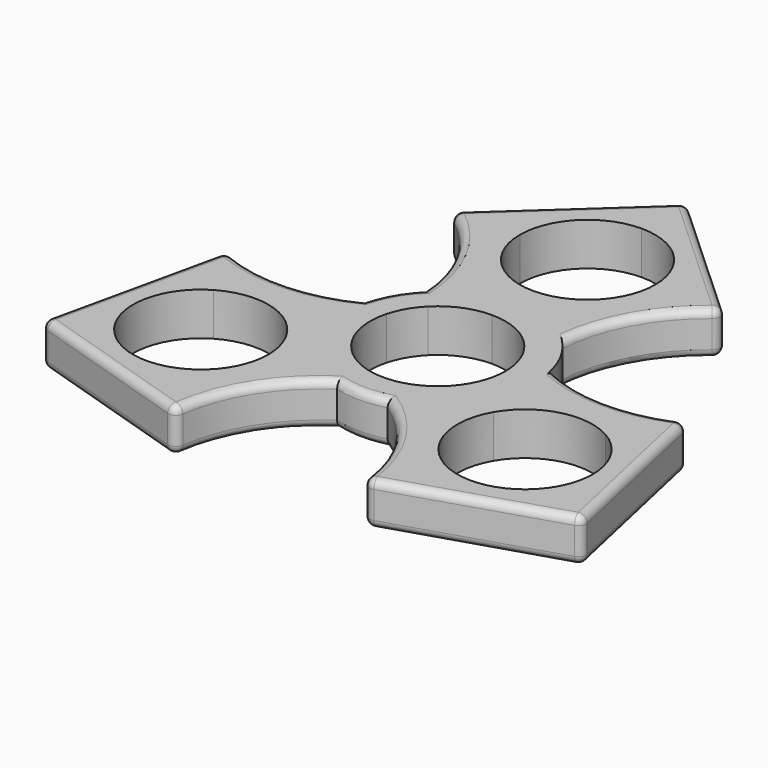
from build123d import *

# Parameters (mm, degrees)
F1_DEPTH      = 6.985
F2_R          = 1.27
F3_T3_DEPTH   = 27.3566440137
F3_T6_ANGLE   = 55.4439181523
F3_S7_R       = 15.875
F3_T8_DEPTH   = 16
F3_T11_DEPTH  = 27.3566440137
F3_T14_DEPTH  = 27.3566440137
F3_T17_ANGLE  = 55.4439181523
F3_S18_R      = 15.875
F3_T19_DEPTH  = 16
F3_T22_ANGLE  = 52.919334491
F3_S23_R      = 25.4
F3_T24_DEPTH  = 10
F3_S25_R      = 25.4
F3_T26_DEPTH  = 10
F3_T29_ANGLE  = 55.4439181523
F3_S30_R      = 15.875
F3_T31_DEPTH  = 15
F3_T34_DEPTH  = 27.3566440137
F3_T37_ANGLE  = 55.4439181523
F3_S38_R      = 15.875
F3_T39_DEPTH  = 16
F3_T42_ANGLE  = 55.4439181523
F3_S43_R      = 15.875
F3_T44_DEPTH  = 15
F3_T47_DEPTH  = 27.3566440137
F3_T50_DEPTH  = 27.3566440137
F3_T53_ANGLE  = 55.4439181523
F3_S54_R      = 15.875
F3_T55_DEPTH  = 16
F3_T58_ANGLE  = 52.919334491
F3_S59_R      = 25.4
F3_T60_DEPTH  = 9
F3_S61_R      = 25.4
F3_T62_DEPTH  = 9
F3_T65_DEPTH  = 27.3566440137
F3_T68_DEPTH  = 27.3566440137
F3_T71_ANGLE  = 55.4439181523
F3_S72_R      = 15.875
F3_T73_DEPTH  = 16
F3_T76_ANGLE  = 52.919334491
F3_S77_R      = 25.4
F3_T78_DEPTH  = 10
F3_S79_R      = 25.4
F3_T80_DEPTH  = 10
F3_T83_ANGLE  = 55.4439181523
F3_S84_R      = 15.875
F3_T85_DEPTH  = 15
F3_T88_DEPTH  = 27.3566440137
F3_T91_DEPTH  = 27.3566440137
F3_T94_ANGLE  = 55.4439181523
F3_S95_R      = 15.875
F3_T96_DEPTH  = 16
F3_T99_ANGLE  = 52.919334491
F3_S100_R     = 25.4
F3_T101_DEPTH = 10
F3_S102_R     = 25.4
F3_T103_DEPTH = 10
F3_T106_ANGLE = 55.4439181523
F3_S107_R     = 15.875
F3_T108_DEPTH = 15
F3_T111_DEPTH = 27.3566440137
F3_T114_DEPTH = 27.3566440137
F3_T117_ANGLE = 55.4439181523
F3_S118_R     = 15.875
F3_T119_DEPTH = 16
F3_T122_ANGLE = 52.919334491
F3_S123_R     = 25.4
F3_T124_DEPTH = 9
F3_S125_R     = 25.4
F3_T126_DEPTH = 9
F3_T129_ANGLE = 55.4439181523
F3_S130_R     = 15.875
F3_T131_DEPTH = 16
F3_T134_ANGLE = 99.5162059051
F3_T137_ANGLE = 99.5162059051
F3_T140_ANGLE = 85.0357607308
F3_T143_ANGLE = 99.5162059051
F3_T146_ANGLE = 99.5162059051
F3_T149_ANGLE = 85.0357607308
F3_T152_ANGLE = 99.5162059051
F3_T155_ANGLE = 99.5162059051
F3_T158_ANGLE = 85.0357607308
F3_T161_ANGLE = 99.5162059051
F3_T164_ANGLE = 85.0357607308
F3_T167_ANGLE = 99.5162059051
F3_T170_ANGLE = 99.5162059051
F3_T173_ANGLE = 85.0357607308
F3_T176_ANGLE = 99.5162059051
F3_T179_ANGLE = 99.5162059051
F3_T182_ANGLE = 85.0357607308
F3_T185_ANGLE = 99.5162059051
F3_T189_ANGLE = 52.919334491
F3_S190_R     = 25.4
F3_T191_DEPTH = 9
F3_T194_ANGLE = 55.4439181523
F3_S195_R     = 15.875
F3_T196_DEPTH = 16
F3_T201_ANGLE = 52.919334491
F3_S202_R     = 25.4
F3_T203_DEPTH = 10
F3_T206_ANGLE = 55.4439181523
F3_S207_R     = 15.875
F3_T208_DEPTH = 16
F3_T213_ANGLE = 55.4439181523
F3_S214_R     = 15.875
F3_T215_DEPTH = 15
F3_T218_ANGLE = 52.919334491
F3_S219_R     = 25.4
F3_T220_DEPTH = 10
F3_T225_ANGLE = 55.4439181523
F3_S226_R     = 15.875
F3_T227_DEPTH = 16
F3_T230_ANGLE = 52.919334491
F3_S231_R     = 25.4
F3_T232_DEPTH = 9
F3_T237_ANGLE = 52.919334491
F3_S238_R     = 25.4
F3_T239_DEPTH = 10
F3_T242_ANGLE = 55.4439181523
F3_S243_R     = 15.875
F3_T244_DEPTH = 16
F3_T249_ANGLE = 55.4439181523
F3_S250_R     = 15.875
F3_T251_DEPTH = 15
F3_T254_ANGLE = 52.919334491
F3_S255_R     = 25.4
F3_T256_DEPTH = 10
F3_T261_ANGLE = 52.919334491
F3_S262_R     = 25.4
F3_T263_DEPTH = 10
F3_T266_ANGLE = 55.4439181523
F3_S267_R     = 15.875
F3_T268_DEPTH = 16
F3_T273_ANGLE = 55.4439181523
F3_S274_R     = 15.875
F3_T275_DEPTH = 15
F3_T278_ANGLE = 52.919334491
F3_S279_R     = 25.4
F3_T280_DEPTH = 10
F3_T285_ANGLE = 55.4439181523
F3_S286_R     = 15.875
F3_T287_DEPTH = 16
F3_T290_ANGLE = 52.919334491
F3_S291_R     = 25.4
F3_T292_DEPTH = 9
F3_T297_ANGLE = 52.919334491
F3_S298_R     = 25.4
F3_T299_DEPTH = 9
F3_T302_ANGLE = 55.4439181523
F3_S303_R     = 15.875
F3_T304_DEPTH = 16


# Not quite as in the source:
# - a fillet or chamfer that OpenCascade refuses, or shapes differently, is made with other operations: its cross-section is extruded or revolved along the edge and cut away or added


with BuildPart() as f1:
    # F0 (on Top) → F1 (new body)
    with BuildSketch(Plane.XY):
        with BuildLine():
            ThreePointArc((10.6357126807, 2.8498306237), (10.9167002241, 1.4372108499), (11.0109, 0))
            ThreePointArc((11.0109, 0), (10.6357126807, -2.8498306237), (9.5357191185, -5.50545))
            Line((9.5357191185, -5.50545), (13.7481532851, -7.9375))
            ThreePointArc((13.7481532851, -7.9375), (15.3340724923, -4.108752341), (15.875, 0))
            ThreePointArc((15.875, 0), (15.7391871743, 2.0721033015), (15.3340724923, 4.108752341))
            Line((15.3340724923, 4.108752341), (10.6357126807, 2.8498306237))
        make_face()
        with BuildLine():
            ThreePointArc((7.785882057, 7.785882057), (9.5357191185, 5.50545), (10.6357126807, 2.8498306237))
            Line((10.6357126807, 2.8498306237), (15.3340724923, 4.108752341))
            ThreePointArc((15.3340724923, 4.108752341), (13.7481532851, 7.9375), (11.2253201513, 11.2253201513))
            Line((11.2253201513, 11.2253201513), (7.785882057, 7.785882057))
        make_face()
        with BuildLine():
            Line((13.7481532851, -7.9375), (9.5357191185, -5.50545))
            ThreePointArc((9.5357191185, -5.50545), (6.7030112187, -8.7355342946), (2.8498306237, -10.6357126807))
            Line((2.8498306237, -10.6357126807), (4.108752341, -15.3340724923))
            ThreePointArc((4.108752341, -15.3340724923), (9.6640876855, -12.5944842771), (13.7481532851, -7.9375))
        make_face()
        with BuildLine():
            ThreePointArc((0, 11.0109), (4.2136890054, 10.1727451445), (7.785882057, 7.785882057))
            Line((7.785882057, 7.785882057), (11.2253201513, 11.2253201513))
            ThreePointArc((11.2253201513, 11.2253201513), (6.0750994888, 14.6665875786), (0, 15.875))
            Line((0, 15.875), (0, 11.0109))
        make_face()
        with BuildLine():
            ThreePointArc((37.4772043073, 3.952421986), (26.387705649, 1.4905349479), (15.3340724923, 4.108752341))
            ThreePointArc((15.3340724923, 4.108752341), (15.7391871743, 2.0721033015), (15.875, 0))
            ThreePointArc((15.875, 0), (15.3340724923, -4.108752341), (13.7481532851, -7.9375))
            Line((13.7481532851, -7.9375), (16.8607351888, -9.73455))
            ThreePointArc((16.8607351888, -9.73455), (23.5466236836, -4.6042873193), (31.9019043073, -5.7042808815))
            Line((31.9019043073, -5.7042808815), (37.4772043073, 3.952421986))
        make_face()
        with BuildLine():
            Line((4.108752341, -15.3340724923), (2.8498306237, -10.6357126807))
            ThreePointArc((2.8498306237, -10.6357126807), (0, -11.0109), (-2.8498306237, -10.6357126807))
            Line((-2.8498306237, -10.6357126807), (-4.108752341, -15.3340724923))
            ThreePointArc((-4.108752341, -15.3340724923), (0, -15.875), (4.108752341, -15.3340724923))
        make_face()
        with BuildLine():
            Line((16.8607351888, -9.73455), (13.7481532851, -7.9375))
            ThreePointArc((13.7481532851, -7.9375), (9.6640876855, -12.5944842771), (4.108752341, -15.3340724923))
            ThreePointArc((4.108752341, -15.3340724923), (11.9030116944, -23.5976909136), (15.3157043073, -34.432421986))
            Line((15.3157043073, -34.432421986), (20.8910043073, -24.7757191185))
            ThreePointArc((20.8910043073, -24.7757191185), (15.7607416267, -18.0898306237), (16.8607351888, -9.73455))
        make_face()
        with BuildLine():
            ThreePointArc((-7.785882057, 7.785882057), (-4.2136890054, 10.1727451445), (0, 11.0109))
            Line((0, 11.0109), (0, 15.875))
            ThreePointArc((0, 15.875), (-6.0750994888, 14.6665875786), (-11.2253201513, 11.2253201513))
            Line((-11.2253201513, 11.2253201513), (-7.785882057, 7.785882057))
        make_face()
        with BuildLine():
            ThreePointArc((0, 15.875), (6.0750994888, 14.6665875786), (11.2253201513, 11.2253201513))
            ThreePointArc((11.2253201513, 11.2253201513), (14.4846939546, 22.1071559657), (22.1615, 30.48))
            Line((22.1615, 30.48), (11.0109, 30.48))
            ThreePointArc((11.0109, 30.48), (7.785882057, 22.694117943), (0, 19.4691))
            Line((0, 19.4691), (0, 15.875))
        make_face()
        with BuildLine():
            Line((-13.7481532851, -7.9375), (-9.5357191185, -5.50545))
            ThreePointArc((-9.5357191185, -5.50545), (-10.9167002241, -1.4372108499), (-10.6357126807, 2.8498306237))
            Line((-10.6357126807, 2.8498306237), (-15.3340724923, 4.108752341))
            ThreePointArc((-15.3340724923, 4.108752341), (-15.7391871743, -2.0721033015), (-13.7481532851, -7.9375))
        make_face()
        with BuildLine():
            ThreePointArc((-2.8498306237, -10.6357126807), (-6.7030112187, -8.7355342946), (-9.5357191185, -5.50545))
            Line((-9.5357191185, -5.50545), (-13.7481532851, -7.9375))
            ThreePointArc((-13.7481532851, -7.9375), (-9.6640876855, -12.5944842771), (-4.108752341, -15.3340724923))
            Line((-4.108752341, -15.3340724923), (-2.8498306237, -10.6357126807))
        make_face()
        with BuildLine():
            ThreePointArc((-10.6357126807, 2.8498306237), (-9.5357191185, 5.50545), (-7.785882057, 7.785882057))
            Line((-7.785882057, 7.785882057), (-11.2253201513, 11.2253201513))
            ThreePointArc((-11.2253201513, 11.2253201513), (-13.7481532851, 7.9375), (-15.3340724923, 4.108752341))
            Line((-15.3340724923, 4.108752341), (-10.6357126807, 2.8498306237))
        make_face()
        with BuildLine():
            Line((43.9940905122, -25.4), (37.4772043073, 3.952421986))
            Line((37.4772043073, 3.952421986), (31.9019043073, -5.7042808815))
            ThreePointArc((31.9019043073, -5.7042808815), (35.9321734259, -9.73455), (37.4073543073, -15.24))
            ThreePointArc((37.4073543073, -15.24), (37.032166988, -18.0898306237), (35.9321734259, -20.74545))
            Line((35.9321734259, -20.74545), (43.9940905122, -25.4))
        make_face()
        with BuildLine():
            ThreePointArc((-11.2253201513, 11.2253201513), (-6.0750994888, 14.6665875786), (0, 15.875))
            Line((0, 15.875), (0, 19.4691))
            ThreePointArc((0, 19.4691), (-7.785882057, 22.694117943), (-11.0109, 30.48))
            Line((-11.0109, 30.48), (-22.1615, 30.48))
            ThreePointArc((-22.1615, 30.48), (-14.4846939546, 22.1071559657), (-11.2253201513, 11.2253201513))
        make_face()
        with BuildLine():
            Line((11.0109, 30.48), (22.1615, 30.48))
            Line((22.1615, 30.48), (0, 50.8))
            Line((0, 50.8), (0, 41.4909))
            ThreePointArc((0, 41.4909), (7.785882057, 38.265882057), (11.0109, 30.48))
        make_face()
        with BuildLine():
            ThreePointArc((-4.108752341, -15.3340724923), (-9.6640876855, -12.5944842771), (-13.7481532851, -7.9375))
            Line((-13.7481532851, -7.9375), (-16.8607351888, -9.73455))
            ThreePointArc((-16.8607351888, -9.73455), (-15.7607416267, -12.3901693763), (-15.3855543073, -15.24))
            ThreePointArc((-15.3855543073, -15.24), (-16.8607351888, -20.74545), (-20.8910043073, -24.7757191185))
            Line((-20.8910043073, -24.7757191185), (-15.3157043073, -34.432421986))
            ThreePointArc((-15.3157043073, -34.432421986), (-11.9030116944, -23.5976909136), (-4.108752341, -15.3340724923))
        make_face()
        with BuildLine():
            Line((-16.8607351888, -9.73455), (-13.7481532851, -7.9375))
            ThreePointArc((-13.7481532851, -7.9375), (-15.7391871743, -2.0721033015), (-15.3340724923, 4.108752341))
            ThreePointArc((-15.3340724923, 4.108752341), (-26.387705649, 1.4905349479), (-37.4772043073, 3.952421986))
            Line((-37.4772043073, 3.952421986), (-31.9019043073, -5.7042808815))
            ThreePointArc((-31.9019043073, -5.7042808815), (-23.5466236836, -4.6042873193), (-16.8607351888, -9.73455))
        make_face()
        with BuildLine():
            Line((15.3157043073, -34.432421986), (43.9940905122, -25.4))
            Line((43.9940905122, -25.4), (35.9321734259, -20.74545))
            ThreePointArc((35.9321734259, -20.74545), (29.2462849311, -25.8757126807), (20.8910043073, -24.7757191185))
            Line((20.8910043073, -24.7757191185), (15.3157043073, -34.432421986))
        make_face()
        with BuildLine():
            Line((0, 41.4909), (0, 50.8))
            Line((0, 50.8), (-22.1615, 30.48))
            Line((-22.1615, 30.48), (-11.0109, 30.48))
            ThreePointArc((-11.0109, 30.48), (-7.785882057, 38.265882057), (0, 41.4909))
        make_face()
        with BuildLine():
            Line((-31.9019043073, -5.7042808815), (-37.4772043073, 3.952421986))
            Line((-37.4772043073, 3.952421986), (-43.9940905122, -25.4))
            Line((-43.9940905122, -25.4), (-35.9321734259, -20.74545))
            ThreePointArc((-35.9321734259, -20.74545), (-37.032166988, -12.3901693763), (-31.9019043073, -5.7042808815))
        make_face()
        with BuildLine():
            Line((-43.9940905122, -25.4), (-15.3157043073, -34.432421986))
            Line((-15.3157043073, -34.432421986), (-20.8910043073, -24.7757191185))
            ThreePointArc((-20.8910043073, -24.7757191185), (-29.2462849311, -25.8757126807), (-35.9321734259, -20.74545))
            Line((-35.9321734259, -20.74545), (-43.9940905122, -25.4))
        make_face()
    extrude(amount=F1_DEPTH)

    # F2
    f2_edges = [f1.edges().sort_by_distance(p)[0] for p in [
        (22.1615, 30.48, 3.4925),
        (0, 50.8, 3.4925),
        (-22.1615, 30.48, 3.4925),
        (37.477204, 3.952422, 3.4925),
        (43.994091, -25.4, 3.4925),
        (15.315704, -34.432422, 3.4925),
        (-15.315704, -34.432422, 3.4925),
        (-43.994091, -25.4, 3.4925),
        (-37.477204, 3.952422, 3.4925),
    ]]
    fillet(f2_edges, radius=F2_R)

    # F3: fillet of radius 1.27 on 29 edges, made by hand


with BuildPart() as f3_tool1:
    # F3_s2 → F3_t3 (new body)
    with BuildSketch(Plane(origin=(24.4464303747, 22.4150651, 0), x_dir=(0, 0, 1), z_dir=(-0.7370664686, -0.6758202578, 0))):
        with BuildLine():
            ThreePointArc((6.985, 36.1729766066), (6.6130256121, 37.0710022187), (5.715, 37.4429766066))
            Line((5.715, 37.4429766066), (6.985, 37.4429766066))
            Line((6.985, 37.4429766066), (6.985, 36.1729766066))
        make_face()
    extrude(amount=F3_T3_DEPTH)


with BuildPart() as f3_tool4:
    # F3_s5 → F3_t6 (revolve)
    with BuildSketch(Plane(origin=(-4.8108803435, -34.3795852428, 0), x_dir=(0, 0, 1), z_dir=(-0.1385839484, -0.99035069, 0))):
        with BuildLine():
            ThreePointArc((6.985, 11.7109494398), (6.6130256121, 10.8129238277), (5.715, 10.4409494398))
            Line((5.715, 10.4409494398), (6.985, 10.4409494398))
            Line((6.985, 10.4409494398), (6.985, 11.7109494398))
        make_face()
    revolve(axis=Axis((10.003825701, -36.452669534, 6.985), (0, 0, -1)), revolution_arc=F3_T6_ANGLE)

    # F3_s7 → F3_t8 (cut, symmetric)
    with BuildSketch(Plane.XY.offset(6.3)):
        Circle(F3_S7_R)
    extrude(amount=F3_T8_DEPTH, both=True, mode=Mode.SUBTRACT)


with BuildPart() as f3_tool9:
    # F3_s10 → F3_t11 (new body)
    with BuildSketch(Plane(origin=(-31.6352309914, 9.9636971863, 0), x_dir=(0, 0, 1), z_dir=(0.9538107459, -0.3004081572, 0))):
        with BuildLine():
            ThreePointArc((6.985, 36.1729766066), (6.6130256121, 37.0710022187), (5.715, 37.4429766066))
            Line((5.715, 37.4429766066), (6.985, 37.4429766066))
            Line((6.985, 37.4429766066), (6.985, 36.1729766066))
        make_face()
    extrude(amount=F3_T11_DEPTH)


with BuildPart() as f3_tool12:
    # F3_s13 → F3_t14 (new body)
    with BuildSketch(Plane(origin=(-1.2594045804, -5.672429061, 0), x_dir=(0, 0, 1), z_dir=(-0.2167442773, -0.976228415, 0))):
        with BuildLine():
            ThreePointArc((6.985, 36.1729766066), (6.6130256121, 37.0710022187), (5.715, 37.4429766066))
            Line((5.715, 37.4429766066), (6.985, 37.4429766066))
            Line((6.985, 37.4429766066), (6.985, 36.1729766066))
        make_face()
    extrude(amount=F3_T14_DEPTH)


with BuildPart() as f3_tool15:
    # F3_s16 → F3_t17 (revolve)
    with BuildSketch(Plane(origin=(-6.1527076501, -4.0584782097, 0), x_dir=(0, 0, 1), z_dir=(0.8347533892, 0.5506239908, 0))):
        with BuildLine():
            ThreePointArc((6.985, -10.4048781253), (6.6130256121, -11.3029037374), (5.715, -11.6748781253))
            Line((5.715, -11.6748781253), (6.985, -11.6748781253))
            Line((6.985, -11.6748781253), (6.985, -10.4048781253))
        make_face()
    revolve(axis=Axis((-26.5670250017, 26.8899019591, 6.985), (0, 0, -1)), revolution_arc=F3_T17_ANGLE)

    # F3_s18 → F3_t19 (cut, symmetric)
    with BuildSketch(Plane.XY.offset(6.3)):
        Circle(F3_S18_R)
    extrude(amount=F3_T19_DEPTH, both=True, mode=Mode.SUBTRACT)


with BuildPart() as f3_tool20:
    # F3_s21 → F3_t22 (revolve)
    with BuildSketch(Plane(origin=(0, 0, 0), x_dir=(0, 0, 1), z_dir=(0.8334970853, 0.5525238536, 0))):
        with BuildLine():
            ThreePointArc((6.985, -14.605), (6.6130256121, -15.5030256121), (5.715, -15.875))
            Line((5.715, -15.875), (6.985, -15.875))
            Line((6.985, -15.875), (6.985, -14.605))
        make_face()
    revolve(axis=Axis((0, 0, 6.985), (0, 0, 1)), revolution_arc=F3_T22_ANGLE)

    # F3_s23 → F3_t24 (intersect, symmetric)
    with BuildSketch(Plane.XY.offset(5.9)):
        with Locations((-36.5708507027, 9.5627675749)):
            Circle(F3_S23_R)
    extrude(amount=F3_T24_DEPTH, both=True, mode=Mode.INTERSECT)

    # F3_s25 → F3_t26 (intersect, symmetric)
    with BuildSketch(Plane.XY.offset(5.9)):
        with Locations((-26.5670250017, 26.8899019591)):
            Circle(F3_S25_R)
    extrude(amount=F3_T26_DEPTH, both=True, mode=Mode.INTERSECT)


with BuildPart() as f3_tool27:
    # F3_s28 → F3_t29 (revolve)
    with BuildSketch(Plane(origin=(-27.3681540201, 21.3561372134, 0), x_dir=(0, 0, 1), z_dir=(-0.788376882, 0.6151925649, 0))):
        with BuildLine():
            ThreePointArc((6.985, 11.7109494398), (6.6130256121, 10.8129238277), (5.715, 10.4409494398))
            Line((5.715, 10.4409494398), (6.985, 10.4409494398))
            Line((6.985, 10.4409494398), (6.985, 11.7109494398))
        make_face()
    revolve(axis=Axis((-36.5708507027, 9.5627675749, 6.985), (0, 0, -1)), revolution_arc=F3_T29_ANGLE)

    # F3_s30 → F3_t31 (cut, symmetric)
    with BuildSketch(Plane.XY.offset(5.9)):
        Circle(F3_S30_R)
    extrude(amount=F3_T31_DEPTH, both=True, mode=Mode.SUBTRACT)


with BuildPart() as f3_tool32:
    # F3_s33 → F3_t34 (new body)
    with BuildSketch(Plane(origin=(-4.2827653778, 3.9268908908, 0), x_dir=(0, 0, 1), z_dir=(-0.7370664686, 0.6758202578, 0))):
        with BuildLine():
            ThreePointArc((6.985, 36.1729766066), (6.6130256121, 37.0710022187), (5.715, 37.4429766066))
            Line((5.715, 37.4429766066), (6.985, 37.4429766066))
            Line((6.985, 37.4429766066), (6.985, 36.1729766066))
        make_face()
    extrude(amount=F3_T34_DEPTH)


with BuildPart() as f3_tool35:
    # F3_s36 → F3_t37 (revolve)
    with BuildSketch(Plane(origin=(-0.4383914053, 7.3576402319, 0), x_dir=(0, 0, 1), z_dir=(0.0594776694, -0.9982296363, 0))):
        with BuildLine():
            ThreePointArc((6.985, -10.4048781253), (6.6130256121, -11.3029037374), (5.715, -11.6748781253))
            Line((5.715, -11.6748781253), (6.985, -11.6748781253))
            Line((6.985, -11.6748781253), (6.985, -10.4048781253))
        make_face()
    revolve(axis=Axis((36.5708507027, 9.5627675749, 6.985), (0, 0, -1)), revolution_arc=F3_T37_ANGLE)

    # F3_s38 → F3_t39 (cut, symmetric)
    with BuildSketch(Plane.XY.offset(6.3)):
        Circle(F3_S38_R)
    extrude(amount=F3_T39_DEPTH, both=True, mode=Mode.SUBTRACT)


with BuildPart() as f3_tool40:
    # F3_s41 → F3_t42 (revolve)
    with BuildSketch(Plane(origin=(32.1790343636, 13.0234480294, 0), x_dir=(0, 0, 1), z_dir=(0.9269608304, 0.3751581251, 0))):
        with BuildLine():
            ThreePointArc((5.715, 10.4409494398), (6.6130256121, 10.8129238277), (6.985, 11.7109494398))
            Line((6.985, 11.7109494398), (6.985, 10.4409494398))
            Line((6.985, 10.4409494398), (5.715, 10.4409494398))
        make_face()
    revolve(axis=Axis((26.5670250017, 26.8899019591, 6.985), (0, 0, -1)), revolution_arc=F3_T42_ANGLE)

    # F3_s43 → F3_t44 (cut, symmetric)
    with BuildSketch(Plane.XY.offset(5.9)):
        Circle(F3_S43_R)
    extrude(amount=F3_T44_DEPTH, both=True, mode=Mode.SUBTRACT)


with BuildPart() as f3_tool45:
    # F3_s46 → F3_t47 (new body)
    with BuildSketch(Plane(origin=(7.1888006167, -32.3787622863, 0), x_dir=(0, 0, 1), z_dir=(-0.2167442773, 0.976228415, 0))):
        with BuildLine():
            ThreePointArc((6.985, 36.1729766066), (6.6130256121, 37.0710022187), (5.715, 37.4429766066))
            Line((5.715, 37.4429766066), (6.985, 37.4429766066))
            Line((6.985, 37.4429766066), (6.985, 36.1729766066))
        make_face()
    extrude(amount=F3_T47_DEPTH)


with BuildPart() as f3_tool48:
    # F3_s49 → F3_t50 (new body)
    with BuildSketch(Plane(origin=(5.5421699582, 1.7455381702, 0), x_dir=(0, 0, 1), z_dir=(0.9538107459, 0.3004081572, 0))):
        with BuildLine():
            ThreePointArc((6.985, 36.1729766066), (6.6130256121, 37.0710022187), (5.715, 37.4429766066))
            Line((5.715, 37.4429766066), (6.985, 37.4429766066))
            Line((6.985, 37.4429766066), (6.985, 36.1729766066))
        make_face()
    extrude(amount=F3_T50_DEPTH)


with BuildPart() as f3_tool51:
    # F3_s52 → F3_t53 (revolve)
    with BuildSketch(Plane(origin=(6.5910990554, -3.2991620222, 0), x_dir=(0, 0, 1), z_dir=(-0.8942310586, 0.4476056455, 0))):
        with BuildLine():
            ThreePointArc((6.985, -10.4048781253), (6.6130256121, -11.3029037374), (5.715, -11.6748781253))
            Line((5.715, -11.6748781253), (6.985, -11.6748781253))
            Line((6.985, -11.6748781253), (6.985, -10.4048781253))
        make_face()
    revolve(axis=Axis((-10.003825701, -36.452669534, 6.985), (0, 0, -1)), revolution_arc=F3_T53_ANGLE)

    # F3_s54 → F3_t55 (cut, symmetric)
    with BuildSketch(Plane.XY.offset(5.9)):
        Circle(F3_S54_R)
    extrude(amount=F3_T55_DEPTH, both=True, mode=Mode.SUBTRACT)


with BuildPart() as f3_tool56:
    # F3_s57 → F3_t58 (revolve)
    with BuildSketch(Plane(origin=(0, 0, 0), x_dir=(0, 0, 1), z_dir=(-0.895248236, 0.4455677231, 0))):
        with BuildLine():
            ThreePointArc((6.985, -14.605), (6.6130256121, -15.5030256121), (5.715, -15.875))
            Line((5.715, -15.875), (6.985, -15.875))
            Line((6.985, -15.875), (6.985, -14.605))
        make_face()
    revolve(axis=Axis((0, 0, 6.985), (0, 0, 1)), revolution_arc=F3_T58_ANGLE)

    # F3_s59 → F3_t60 (intersect, symmetric)
    with BuildSketch(Plane.XY.offset(5.9)):
        with Locations((-10.003825701, -36.452669534)):
            Circle(F3_S59_R)
    extrude(amount=F3_T60_DEPTH, both=True, mode=Mode.INTERSECT)

    # F3_s61 → F3_t62 (intersect, symmetric)
    with BuildSketch(Plane.XY.offset(5.9)):
        with Locations((10.003825701, -36.452669534)):
            Circle(F3_S61_R)
    extrude(amount=F3_T62_DEPTH, both=True, mode=Mode.INTERSECT)


with BuildPart() as f3_tool63:
    # F3_s64 → F3_t65 (new body)
    with BuildSketch(Plane(origin=(-31.6352309914, 9.9636971863, 0), x_dir=(0, 0, 1), z_dir=(0.9538107459, -0.3004081572, 0))):
        with BuildLine():
            ThreePointArc((0, 36.1729766066), (0.3719743879, 37.0710022187), (1.27, 37.4429766066))
            Line((1.27, 37.4429766066), (0, 37.4429766066))
            Line((0, 37.4429766066), (0, 36.1729766066))
        make_face()
    extrude(amount=F3_T65_DEPTH)


with BuildPart() as f3_tool66:
    # F3_s67 → F3_t68 (new body)
    with BuildSketch(Plane(origin=(-1.2594045804, -5.672429061, 0), x_dir=(0, 0, 1), z_dir=(-0.2167442773, -0.976228415, 0))):
        with BuildLine():
            ThreePointArc((0, 36.1729766066), (0.3719743879, 37.0710022187), (1.27, 37.4429766066))
            Line((1.27, 37.4429766066), (0, 37.4429766066))
            Line((0, 37.4429766066), (0, 36.1729766066))
        make_face()
    extrude(amount=F3_T68_DEPTH)


with BuildPart() as f3_tool69:
    # F3_s70 → F3_t71 (revolve)
    with BuildSketch(Plane(origin=(-6.1527076501, -4.0584782097, 0), x_dir=(0, 0, 1), z_dir=(0.8347533892, 0.5506239908, 0))):
        with BuildLine():
            ThreePointArc((0, -10.4048781253), (0.3719743879, -11.3029037374), (1.27, -11.6748781253))
            Line((1.27, -11.6748781253), (0, -11.6748781253))
            Line((0, -11.6748781253), (0, -10.4048781253))
        make_face()
    revolve(axis=Axis((-26.5670250017, 26.8899019591, 0), (0, 0, -1)), revolution_arc=F3_T71_ANGLE)

    # F3_s72 → F3_t73 (cut, symmetric)
    with BuildSketch(Plane.XY.offset(0.6)):
        Circle(F3_S72_R)
    extrude(amount=F3_T73_DEPTH, both=True, mode=Mode.SUBTRACT)


with BuildPart() as f3_tool74:
    # F3_s75 → F3_t76 (revolve)
    with BuildSketch(Plane(origin=(0, 0, 0), x_dir=(0, 0, 1), z_dir=(0.8334970853, 0.5525238536, 0))):
        with BuildLine():
            ThreePointArc((0, -14.605), (0.3719743879, -15.5030256121), (1.27, -15.875))
            Line((1.27, -15.875), (0, -15.875))
            Line((0, -15.875), (0, -14.605))
        make_face()
    revolve(axis=Axis((0, 0, 0), (0, 0, 1)), revolution_arc=F3_T76_ANGLE)

    # F3_s77 → F3_t78 (intersect, symmetric)
    with BuildSketch(Plane.XY.offset(1.1)):
        with Locations((-36.5708507027, 9.5627675749)):
            Circle(F3_S77_R)
    extrude(amount=F3_T78_DEPTH, both=True, mode=Mode.INTERSECT)

    # F3_s79 → F3_t80 (intersect, symmetric)
    with BuildSketch(Plane.XY.offset(1.1)):
        with Locations((-26.5670250017, 26.8899019591)):
            Circle(F3_S79_R)
    extrude(amount=F3_T80_DEPTH, both=True, mode=Mode.INTERSECT)


with BuildPart() as f3_tool81:
    # F3_s82 → F3_t83 (revolve)
    with BuildSketch(Plane(origin=(-27.3681540201, 21.3561372134, 0), x_dir=(0, 0, 1), z_dir=(-0.788376882, 0.6151925649, 0))):
        with BuildLine():
            ThreePointArc((0, 11.7109494398), (0.3719743879, 10.8129238277), (1.27, 10.4409494398))
            Line((1.27, 10.4409494398), (0, 10.4409494398))
            Line((0, 10.4409494398), (0, 11.7109494398))
        make_face()
    revolve(axis=Axis((-36.5708507027, 9.5627675749, 0), (0, 0, -1)), revolution_arc=F3_T83_ANGLE)

    # F3_s84 → F3_t85 (cut, symmetric)
    with BuildSketch(Plane.XY.offset(1.1)):
        Circle(F3_S84_R)
    extrude(amount=F3_T85_DEPTH, both=True, mode=Mode.SUBTRACT)


with BuildPart() as f3_tool86:
    # F3_s87 → F3_t88 (new body)
    with BuildSketch(Plane(origin=(24.4464303747, 22.4150651, 0), x_dir=(0, 0, 1), z_dir=(-0.7370664686, -0.6758202578, 0))):
        with BuildLine():
            ThreePointArc((0, 36.1729766066), (0.3719743879, 37.0710022187), (1.27, 37.4429766066))
            Line((1.27, 37.4429766066), (0, 37.4429766066))
            Line((0, 37.4429766066), (0, 36.1729766066))
        make_face()
    extrude(amount=F3_T88_DEPTH)


with BuildPart() as f3_tool89:
    # F3_s90 → F3_t91 (new body)
    with BuildSketch(Plane(origin=(-4.2827653778, 3.9268908908, 0), x_dir=(0, 0, 1), z_dir=(-0.7370664686, 0.6758202578, 0))):
        with BuildLine():
            ThreePointArc((0, 36.1729766066), (0.3719743879, 37.0710022187), (1.27, 37.4429766066))
            Line((1.27, 37.4429766066), (0, 37.4429766066))
            Line((0, 37.4429766066), (0, 36.1729766066))
        make_face()
    extrude(amount=F3_T91_DEPTH)


with BuildPart() as f3_tool92:
    # F3_s93 → F3_t94 (revolve)
    with BuildSketch(Plane(origin=(-0.4383914053, 7.3576402319, 0), x_dir=(0, 0, 1), z_dir=(0.0594776694, -0.9982296363, 0))):
        with BuildLine():
            ThreePointArc((0, -10.4048781253), (0.3719743879, -11.3029037374), (1.27, -11.6748781253))
            Line((1.27, -11.6748781253), (0, -11.6748781253))
            Line((0, -11.6748781253), (0, -10.4048781253))
        make_face()
    revolve(axis=Axis((36.5708507027, 9.5627675749, 0), (0, 0, -1)), revolution_arc=F3_T94_ANGLE)

    # F3_s95 → F3_t96 (cut, symmetric)
    with BuildSketch(Plane.XY.offset(0.6)):
        Circle(F3_S95_R)
    extrude(amount=F3_T96_DEPTH, both=True, mode=Mode.SUBTRACT)


with BuildPart() as f3_tool97:
    # F3_s98 → F3_t99 (revolve)
    with BuildSketch(Plane(origin=(0, 0, 0), x_dir=(0, 0, 1), z_dir=(0.0617511507, -0.9980915767, 0))):
        with BuildLine():
            ThreePointArc((0, -14.605), (0.3719743879, -15.5030256121), (1.27, -15.875))
            Line((1.27, -15.875), (0, -15.875))
            Line((0, -15.875), (0, -14.605))
        make_face()
    revolve(axis=Axis((0, 0, 0), (0, 0, 1)), revolution_arc=F3_T99_ANGLE)

    # F3_s100 → F3_t101 (intersect, symmetric)
    with BuildSketch(Plane.XY.offset(1.1)):
        with Locations((26.5670250017, 26.8899019591)):
            Circle(F3_S100_R)
    extrude(amount=F3_T101_DEPTH, both=True, mode=Mode.INTERSECT)

    # F3_s102 → F3_t103 (intersect, symmetric)
    with BuildSketch(Plane.XY.offset(1.1)):
        with Locations((36.5708507027, 9.5627675749)):
            Circle(F3_S102_R)
    extrude(amount=F3_T103_DEPTH, both=True, mode=Mode.INTERSECT)


with BuildPart() as f3_tool104:
    # F3_s105 → F3_t106 (revolve)
    with BuildSketch(Plane(origin=(32.1790343636, 13.0234480294, 0), x_dir=(0, 0, 1), z_dir=(0.9269608304, 0.3751581251, 0))):
        with BuildLine():
            ThreePointArc((1.27, 10.4409494398), (0.3719743879, 10.8129238277), (0, 11.7109494398))
            Line((0, 11.7109494398), (0, 10.4409494398))
            Line((0, 10.4409494398), (1.27, 10.4409494398))
        make_face()
    revolve(axis=Axis((26.5670250017, 26.8899019591, 0), (0, 0, -1)), revolution_arc=F3_T106_ANGLE)

    # F3_s107 → F3_t108 (cut, symmetric)
    with BuildSketch(Plane.XY.offset(1.1)):
        Circle(F3_S107_R)
    extrude(amount=F3_T108_DEPTH, both=True, mode=Mode.SUBTRACT)


with BuildPart() as f3_tool109:
    # F3_s110 → F3_t111 (new body)
    with BuildSketch(Plane(origin=(7.1888006167, -32.3787622863, 0), x_dir=(0, 0, 1), z_dir=(-0.2167442773, 0.976228415, 0))):
        with BuildLine():
            ThreePointArc((0, 36.1729766066), (0.3719743879, 37.0710022187), (1.27, 37.4429766066))
            Line((1.27, 37.4429766066), (0, 37.4429766066))
            Line((0, 37.4429766066), (0, 36.1729766066))
        make_face()
    extrude(amount=F3_T111_DEPTH)


with BuildPart() as f3_tool112:
    # F3_s113 → F3_t114 (new body)
    with BuildSketch(Plane(origin=(5.5421699582, 1.7455381702, 0), x_dir=(0, 0, 1), z_dir=(0.9538107459, 0.3004081572, 0))):
        with BuildLine():
            ThreePointArc((0, 36.1729766066), (0.3719743879, 37.0710022187), (1.27, 37.4429766066))
            Line((1.27, 37.4429766066), (0, 37.4429766066))
            Line((0, 37.4429766066), (0, 36.1729766066))
        make_face()
    extrude(amount=F3_T114_DEPTH)


with BuildPart() as f3_tool115:
    # F3_s116 → F3_t117 (revolve)
    with BuildSketch(Plane(origin=(6.5910990554, -3.2991620222, 0), x_dir=(0, 0, 1), z_dir=(-0.8942310586, 0.4476056455, 0))):
        with BuildLine():
            ThreePointArc((0, -10.4048781253), (0.3719743879, -11.3029037374), (1.27, -11.6748781253))
            Line((1.27, -11.6748781253), (0, -11.6748781253))
            Line((0, -11.6748781253), (0, -10.4048781253))
        make_face()
    revolve(axis=Axis((-10.003825701, -36.452669534, 0), (0, 0, -1)), revolution_arc=F3_T117_ANGLE)

    # F3_s118 → F3_t119 (cut, symmetric)
    with BuildSketch(Plane.XY.offset(1.1)):
        Circle(F3_S118_R)
    extrude(amount=F3_T119_DEPTH, both=True, mode=Mode.SUBTRACT)


with BuildPart() as f3_tool120:
    # F3_s121 → F3_t122 (revolve)
    with BuildSketch(Plane(origin=(0, 0, 0), x_dir=(0, 0, 1), z_dir=(-0.895248236, 0.4455677231, 0))):
        with BuildLine():
            ThreePointArc((0, -14.605), (0.3719743879, -15.5030256121), (1.27, -15.875))
            Line((1.27, -15.875), (0, -15.875))
            Line((0, -15.875), (0, -14.605))
        make_face()
    revolve(axis=Axis((0, 0, 0), (0, 0, 1)), revolution_arc=F3_T122_ANGLE)

    # F3_s123 → F3_t124 (intersect, symmetric)
    with BuildSketch(Plane.XY.offset(1.1)):
        with Locations((-10.003825701, -36.452669534)):
            Circle(F3_S123_R)
    extrude(amount=F3_T124_DEPTH, both=True, mode=Mode.INTERSECT)

    # F3_s125 → F3_t126 (intersect, symmetric)
    with BuildSketch(Plane.XY.offset(1.1)):
        with Locations((10.003825701, -36.452669534)):
            Circle(F3_S125_R)
    extrude(amount=F3_T126_DEPTH, both=True, mode=Mode.INTERSECT)


with BuildPart() as f3_tool127:
    # F3_s128 → F3_t129 (revolve)
    with BuildSketch(Plane(origin=(-4.8108803435, -34.3795852428, 0), x_dir=(0, 0, 1), z_dir=(-0.1385839484, -0.99035069, 0))):
        with BuildLine():
            ThreePointArc((0, 11.7109494398), (0.3719743879, 10.8129238277), (1.27, 10.4409494398))
            Line((1.27, 10.4409494398), (0, 10.4409494398))
            Line((0, 10.4409494398), (0, 11.7109494398))
        make_face()
    revolve(axis=Axis((10.003825701, -36.452669534, 0), (0, 0, -1)), revolution_arc=F3_T129_ANGLE)

    # F3_s130 → F3_t131 (cut, symmetric)
    with BuildSketch(Plane.XY.offset(0.6)):
        Circle(F3_S130_R)
    extrude(amount=F3_T131_DEPTH, both=True, mode=Mode.SUBTRACT)


with BuildPart() as f3_tool132:
    # F3_s133 → F3_t134 (revolve)
    with BuildSketch(Plane(origin=(-5.5421699582, 1.7455381702, 0), x_dir=(0, 0, 1), z_dir=(-0.9538107459, 0.3004081572, 0))):
        with BuildLine():
            ThreePointArc((0, -36.1729766066), (0.3719743879, -37.0710022187), (1.27, -37.4429766066))
            Line((1.27, -37.4429766066), (0, -37.4429766066))
            Line((0, -37.4429766066), (0, -36.1729766066))
        make_face()
    revolve(axis=Axis((-16.4088272021, -32.7566356298, 0), (0, 0, 1)), revolution_arc=F3_T134_ANGLE)


with BuildPart() as f3_tool135:
    # F3_s136 → F3_t137 (revolve)
    with BuildSketch(Plane(origin=(4.8108803435, -34.3795852428, 0), x_dir=(0, 0, 1), z_dir=(-0.1385839484, 0.99035069, 0))):
        with BuildLine():
            ThreePointArc((0, 11.7109494398), (0.3719743879, 10.8129238277), (1.27, 10.4409494398))
            Line((1.27, 10.4409494398), (0, 10.4409494398))
            Line((0, 10.4409494398), (0, 11.7109494398))
        make_face()
    revolve(axis=Axis((16.4088272021, -32.7566356298, 0), (0, 0, 1)), revolution_arc=F3_T137_ANGLE)


with BuildPart() as f3_tool138:
    # F3_s139 → F3_t140 (revolve)
    with BuildSketch(Plane(origin=(31.6352309914, 9.9636971863, 0), x_dir=(0, 0, 1), z_dir=(-0.9538107459, -0.3004081572, 0))):
        with BuildLine():
            ThreePointArc((0, -36.1729766066), (0.3719743879, -37.0710022187), (1.27, -37.4429766066))
            Line((1.27, -37.4429766066), (0, -37.4429766066))
            Line((0, -37.4429766066), (0, -36.1729766066))
        make_face()
    revolve(axis=Axis((42.5018882352, -24.5384766137, 0), (0, 0, 1)), revolution_arc=F3_T140_ANGLE)


with BuildPart() as f3_tool141:
    # F3_s142 → F3_t143 (revolve)
    with BuildSketch(Plane(origin=(32.1790343636, 13.0234480294, 0), x_dir=(0, 0, 1), z_dir=(-0.9269608304, -0.3751581251, 0))):
        with BuildLine():
            ThreePointArc((0, -11.7109494398), (0.3719743879, -10.8129238277), (1.27, -10.4409494398))
            Line((1.27, -10.4409494398), (0, -10.4409494398))
            Line((0, -10.4409494398), (0, -11.7109494398))
        make_face()
    revolve(axis=Axis((36.5724921989, 2.1678566116, 0), (0, 0, -1)), revolution_arc=F3_T143_ANGLE)


with BuildPart() as f3_tool144:
    # F3_s145 → F3_t146 (revolve)
    with BuildSketch(Plane(origin=(27.3681540201, 21.3561372134, 0), x_dir=(0, 0, 1), z_dir=(-0.788376882, -0.6151925649, 0))):
        with BuildLine():
            ThreePointArc((0, 11.7109494398), (0.3719743879, 10.8129238277), (1.27, 10.4409494398))
            Line((1.27, 10.4409494398), (0, 10.4409494398))
            Line((0, 10.4409494398), (0, 11.7109494398))
        make_face()
    revolve(axis=Axis((20.1636649969, 30.5887790182, 0), (0, 0, 1)), revolution_arc=F3_T146_ANGLE)


with BuildPart() as f3_tool147:
    # F3_s148 → F3_t149 (revolve)
    with BuildSketch(Plane(origin=(-24.4464303747, 22.4150651, 0), x_dir=(0, 0, 1), z_dir=(0.7370664686, -0.6758202578, 0))):
        with BuildLine():
            ThreePointArc((0, -36.1729766066), (0.3719743879, -37.0710022187), (1.27, -37.4429766066))
            Line((1.27, -37.4429766066), (0, -37.4429766066))
            Line((0, -37.4429766066), (0, -36.1729766066))
        make_face()
    revolve(axis=Axis((0, 49.0769532274, 0), (0, 0, 1)), revolution_arc=F3_T149_ANGLE)


with BuildPart() as f3_tool150:
    # F3_s151 → F3_t152 (revolve)
    with BuildSketch(Plane(origin=(4.2827653778, 3.9268908908, 0), x_dir=(0, 0, 1), z_dir=(0.7370664686, 0.6758202578, 0))):
        with BuildLine():
            ThreePointArc((0, -36.1729766066), (0.3719743879, -37.0710022187), (1.27, -37.4429766066))
            Line((1.27, -37.4429766066), (0, -37.4429766066))
            Line((0, -37.4429766066), (0, -36.1729766066))
        make_face()
    revolve(axis=Axis((-20.1636649969, 30.5887790182, 0), (0, 0, 1)), revolution_arc=F3_T152_ANGLE)


with BuildPart() as f3_tool153:
    # F3_s154 → F3_t155 (revolve)
    with BuildSketch(Plane(origin=(-32.1790343636, 13.0234480294, 0), x_dir=(0, 0, 1), z_dir=(0.9269608304, -0.3751581251, 0))):
        with BuildLine():
            ThreePointArc((0, 11.7109494398), (0.3719743879, 10.8129238277), (1.27, 10.4409494398))
            Line((1.27, 10.4409494398), (0, 10.4409494398))
            Line((0, 10.4409494398), (0, 11.7109494398))
        make_face()
    revolve(axis=Axis((-36.5724921989, 2.1678566116, 0), (0, 0, 1)), revolution_arc=F3_T155_ANGLE)


with BuildPart() as f3_tool156:
    # F3_s157 → F3_t158 (revolve)
    with BuildSketch(Plane(origin=(-7.1888006167, -32.3787622863, 0), x_dir=(0, 0, 1), z_dir=(0.2167442773, 0.976228415, 0))):
        with BuildLine():
            ThreePointArc((0, -36.1729766066), (0.3719743879, -37.0710022187), (1.27, -37.4429766066))
            Line((1.27, -37.4429766066), (0, -37.4429766066))
            Line((0, -37.4429766066), (0, -36.1729766066))
        make_face()
    revolve(axis=Axis((-42.5018882352, -24.5384766137, 0), (0, 0, 1)), revolution_arc=F3_T158_ANGLE)


with BuildPart() as f3_tool159:
    # F3_s160 → F3_t161 (revolve)
    with BuildSketch(Plane(origin=(4.8108803435, -34.3795852428, 0), x_dir=(0, 0, 1), z_dir=(-0.1385839484, 0.99035069, 0))):
        with BuildLine():
            ThreePointArc((6.985, 11.7109494398), (6.6130256121, 10.8129238277), (5.715, 10.4409494398))
            Line((5.715, 10.4409494398), (6.985, 10.4409494398))
            Line((6.985, 10.4409494398), (6.985, 11.7109494398))
        make_face()
    revolve(axis=Axis((16.4088272021, -32.7566356298, 6.985), (0, 0, 1)), revolution_arc=F3_T161_ANGLE)


with BuildPart() as f3_tool162:
    # F3_s163 → F3_t164 (revolve)
    with BuildSketch(Plane(origin=(31.6352309914, 9.9636971863, 0), x_dir=(0, 0, 1), z_dir=(-0.9538107459, -0.3004081572, 0))):
        with BuildLine():
            ThreePointArc((6.985, -36.1729766066), (6.6130256121, -37.0710022187), (5.715, -37.4429766066))
            Line((5.715, -37.4429766066), (6.985, -37.4429766066))
            Line((6.985, -37.4429766066), (6.985, -36.1729766066))
        make_face()
    revolve(axis=Axis((42.5018882352, -24.5384766137, 6.985), (0, 0, 1)), revolution_arc=F3_T164_ANGLE)


with BuildPart() as f3_tool165:
    # F3_s166 → F3_t167 (revolve)
    with BuildSketch(Plane(origin=(32.1790343636, 13.0234480294, 0), x_dir=(0, 0, 1), z_dir=(-0.9269608304, -0.3751581251, 0))):
        with BuildLine():
            ThreePointArc((5.715, -10.4409494398), (6.6130256121, -10.8129238277), (6.985, -11.7109494398))
            Line((6.985, -11.7109494398), (6.985, -10.4409494398))
            Line((6.985, -10.4409494398), (5.715, -10.4409494398))
        make_face()
    revolve(axis=Axis((36.5724921989, 2.1678566116, 6.985), (0, 0, -1)), revolution_arc=F3_T167_ANGLE)


with BuildPart() as f3_tool168:
    # F3_s169 → F3_t170 (revolve)
    with BuildSketch(Plane(origin=(27.3681540201, 21.3561372134, 0), x_dir=(0, 0, 1), z_dir=(-0.788376882, -0.6151925649, 0))):
        with BuildLine():
            ThreePointArc((6.985, 11.7109494398), (6.6130256121, 10.8129238277), (5.715, 10.4409494398))
            Line((5.715, 10.4409494398), (6.985, 10.4409494398))
            Line((6.985, 10.4409494398), (6.985, 11.7109494398))
        make_face()
    revolve(axis=Axis((20.1636649969, 30.5887790182, 6.985), (0, 0, 1)), revolution_arc=F3_T170_ANGLE)


with BuildPart() as f3_tool171:
    # F3_s172 → F3_t173 (revolve)
    with BuildSketch(Plane(origin=(-24.4464303747, 22.4150651, 0), x_dir=(0, 0, 1), z_dir=(0.7370664686, -0.6758202578, 0))):
        with BuildLine():
            ThreePointArc((6.985, -36.1729766066), (6.6130256121, -37.0710022187), (5.715, -37.4429766066))
            Line((5.715, -37.4429766066), (6.985, -37.4429766066))
            Line((6.985, -37.4429766066), (6.985, -36.1729766066))
        make_face()
    revolve(axis=Axis((0, 49.0769532274, 6.985), (0, 0, 1)), revolution_arc=F3_T173_ANGLE)


with BuildPart() as f3_tool174:
    # F3_s175 → F3_t176 (revolve)
    with BuildSketch(Plane(origin=(4.2827653778, 3.9268908908, 0), x_dir=(0, 0, 1), z_dir=(0.7370664686, 0.6758202578, 0))):
        with BuildLine():
            ThreePointArc((6.985, -36.1729766066), (6.6130256121, -37.0710022187), (5.715, -37.4429766066))
            Line((5.715, -37.4429766066), (6.985, -37.4429766066))
            Line((6.985, -37.4429766066), (6.985, -36.1729766066))
        make_face()
    revolve(axis=Axis((-20.1636649969, 30.5887790182, 6.985), (0, 0, 1)), revolution_arc=F3_T176_ANGLE)


with BuildPart() as f3_tool177:
    # F3_s178 → F3_t179 (revolve)
    with BuildSketch(Plane(origin=(-32.1790343636, 13.0234480294, 0), x_dir=(0, 0, 1), z_dir=(0.9269608304, -0.3751581251, 0))):
        with BuildLine():
            ThreePointArc((6.985, 11.7109494398), (6.6130256121, 10.8129238277), (5.715, 10.4409494398))
            Line((5.715, 10.4409494398), (6.985, 10.4409494398))
            Line((6.985, 10.4409494398), (6.985, 11.7109494398))
        make_face()
    revolve(axis=Axis((-36.5724921989, 2.1678566116, 6.985), (0, 0, 1)), revolution_arc=F3_T179_ANGLE)


with BuildPart() as f3_tool180:
    # F3_s181 → F3_t182 (revolve)
    with BuildSketch(Plane(origin=(-7.1888006167, -32.3787622863, 0), x_dir=(0, 0, 1), z_dir=(0.2167442773, 0.976228415, 0))):
        with BuildLine():
            ThreePointArc((6.985, -36.1729766066), (6.6130256121, -37.0710022187), (5.715, -37.4429766066))
            Line((5.715, -37.4429766066), (6.985, -37.4429766066))
            Line((6.985, -37.4429766066), (6.985, -36.1729766066))
        make_face()
    revolve(axis=Axis((-42.5018882352, -24.5384766137, 6.985), (0, 0, 1)), revolution_arc=F3_T182_ANGLE)


with BuildPart() as f3_tool183:
    # F3_s184 → F3_t185 (revolve)
    with BuildSketch(Plane(origin=(-5.5421699582, 1.7455381702, 0), x_dir=(0, 0, 1), z_dir=(-0.9538107459, 0.3004081572, 0))):
        with BuildLine():
            ThreePointArc((6.985, -36.1729766066), (6.6130256121, -37.0710022187), (5.715, -37.4429766066))
            Line((5.715, -37.4429766066), (6.985, -37.4429766066))
            Line((6.985, -37.4429766066), (6.985, -36.1729766066))
        make_face()
    revolve(axis=Axis((-16.4088272021, -32.7566356298, 6.985), (0, 0, 1)), revolution_arc=F3_T185_ANGLE)


with BuildPart() as f3_tool187:
    # F3_s188 → F3_t189 (revolve)
    with BuildSketch(Plane(origin=(0, 0, 0), x_dir=(0, 0, 1), z_dir=(-0.895248236, 0.4455677231, 0))):
        with BuildLine():
            ThreePointArc((6.985, -14.605), (6.6130256121, -15.5030256121), (5.715, -15.875))
            Line((5.715, -15.875), (6.985, -15.875))
            Line((6.985, -15.875), (6.985, -14.605))
        make_face()
    revolve(axis=Axis((0, 0, 6.985), (0, 0, 1)), revolution_arc=F3_T189_ANGLE)

    # F3_s190 → F3_t191 (cut, symmetric)
    with BuildSketch(Plane.XY.offset(5.9)):
        with Locations((10.003825701, -36.452669534)):
            Circle(F3_S190_R)
    extrude(amount=F3_T191_DEPTH, both=True, mode=Mode.SUBTRACT)


with BuildPart() as f3_tool192:
    # F3_s193 → F3_t194 (revolve)
    with BuildSketch(Plane(origin=(-4.8108803435, -34.3795852428, 0), x_dir=(0, 0, 1), z_dir=(-0.1385839484, -0.99035069, 0))):
        with BuildLine():
            ThreePointArc((6.985, 11.7109494398), (6.6130256121, 10.8129238277), (5.715, 10.4409494398))
            Line((5.715, 10.4409494398), (6.985, 10.4409494398))
            Line((6.985, 10.4409494398), (6.985, 11.7109494398))
        make_face()
    revolve(axis=Axis((10.003825701, -36.452669534, 6.985), (0, 0, -1)), revolution_arc=F3_T194_ANGLE)

    # F3_s195 → F3_t196 (intersect, symmetric)
    with BuildSketch(Plane.XY.offset(6.3)):
        Circle(F3_S195_R)
    extrude(amount=F3_T196_DEPTH, both=True, mode=Mode.INTERSECT)


with BuildPart() as f3_tool187_1:
    add(f3_tool187.part)

    # F3_t197: intersect F3_tool192
    add(f3_tool192.part, mode=Mode.INTERSECT)


with BuildPart() as f3_tool199:
    # F3_s200 → F3_t201 (revolve)
    with BuildSketch(Plane(origin=(0, 0, 0), x_dir=(0, 0, 1), z_dir=(0.8334970853, 0.5525238536, 0))):
        with BuildLine():
            ThreePointArc((6.985, -14.605), (6.6130256121, -15.5030256121), (5.715, -15.875))
            Line((5.715, -15.875), (6.985, -15.875))
            Line((6.985, -15.875), (6.985, -14.605))
        make_face()
    revolve(axis=Axis((0, 0, 6.985), (0, 0, 1)), revolution_arc=F3_T201_ANGLE)

    # F3_s202 → F3_t203 (cut, symmetric)
    with BuildSketch(Plane.XY.offset(5.9)):
        with Locations((-26.5670250017, 26.8899019591)):
            Circle(F3_S202_R)
    extrude(amount=F3_T203_DEPTH, both=True, mode=Mode.SUBTRACT)


with BuildPart() as f3_tool204:
    # F3_s205 → F3_t206 (revolve)
    with BuildSketch(Plane(origin=(-6.1527076501, -4.0584782097, 0), x_dir=(0, 0, 1), z_dir=(0.8347533892, 0.5506239908, 0))):
        with BuildLine():
            ThreePointArc((6.985, -10.4048781253), (6.6130256121, -11.3029037374), (5.715, -11.6748781253))
            Line((5.715, -11.6748781253), (6.985, -11.6748781253))
            Line((6.985, -11.6748781253), (6.985, -10.4048781253))
        make_face()
    revolve(axis=Axis((-26.5670250017, 26.8899019591, 6.985), (0, 0, -1)), revolution_arc=F3_T206_ANGLE)

    # F3_s207 → F3_t208 (intersect, symmetric)
    with BuildSketch(Plane.XY.offset(6.3)):
        Circle(F3_S207_R)
    extrude(amount=F3_T208_DEPTH, both=True, mode=Mode.INTERSECT)


with BuildPart() as f3_tool199_1:
    add(f3_tool199.part)

    # F3_t209: intersect F3_tool204
    add(f3_tool204.part, mode=Mode.INTERSECT)


with BuildPart() as f3_tool211:
    # F3_s212 → F3_t213 (revolve)
    with BuildSketch(Plane(origin=(-27.3681540201, 21.3561372134, 0), x_dir=(0, 0, 1), z_dir=(-0.788376882, 0.6151925649, 0))):
        with BuildLine():
            ThreePointArc((6.985, 11.7109494398), (6.6130256121, 10.8129238277), (5.715, 10.4409494398))
            Line((5.715, 10.4409494398), (6.985, 10.4409494398))
            Line((6.985, 10.4409494398), (6.985, 11.7109494398))
        make_face()
    revolve(axis=Axis((-36.5708507027, 9.5627675749, 6.985), (0, 0, -1)), revolution_arc=F3_T213_ANGLE)

    # F3_s214 → F3_t215 (intersect, symmetric)
    with BuildSketch(Plane.XY.offset(5.9)):
        Circle(F3_S214_R)
    extrude(amount=F3_T215_DEPTH, both=True, mode=Mode.INTERSECT)


with BuildPart() as f3_tool216:
    # F3_s217 → F3_t218 (revolve)
    with BuildSketch(Plane(origin=(0, 0, 0), x_dir=(0, 0, 1), z_dir=(0.8334970853, 0.5525238536, 0))):
        with BuildLine():
            ThreePointArc((6.985, -14.605), (6.6130256121, -15.5030256121), (5.715, -15.875))
            Line((5.715, -15.875), (6.985, -15.875))
            Line((6.985, -15.875), (6.985, -14.605))
        make_face()
    revolve(axis=Axis((0, 0, 6.985), (0, 0, 1)), revolution_arc=F3_T218_ANGLE)

    # F3_s219 → F3_t220 (cut, symmetric)
    with BuildSketch(Plane.XY.offset(5.9)):
        with Locations((-36.5708507027, 9.5627675749)):
            Circle(F3_S219_R)
    extrude(amount=F3_T220_DEPTH, both=True, mode=Mode.SUBTRACT)


with BuildPart() as f3_tool211_1:
    add(f3_tool211.part)

    # F3_t221: intersect F3_tool216
    add(f3_tool216.part, mode=Mode.INTERSECT)


with BuildPart() as f3_tool223:
    # F3_s224 → F3_t225 (revolve)
    with BuildSketch(Plane(origin=(6.5910990554, -3.2991620222, 0), x_dir=(0, 0, 1), z_dir=(-0.8942310586, 0.4476056455, 0))):
        with BuildLine():
            ThreePointArc((6.985, -10.4048781253), (6.6130256121, -11.3029037374), (5.715, -11.6748781253))
            Line((5.715, -11.6748781253), (6.985, -11.6748781253))
            Line((6.985, -11.6748781253), (6.985, -10.4048781253))
        make_face()
    revolve(axis=Axis((-10.003825701, -36.452669534, 6.985), (0, 0, -1)), revolution_arc=F3_T225_ANGLE)

    # F3_s226 → F3_t227 (intersect, symmetric)
    with BuildSketch(Plane.XY.offset(5.9)):
        Circle(F3_S226_R)
    extrude(amount=F3_T227_DEPTH, both=True, mode=Mode.INTERSECT)


with BuildPart() as f3_tool228:
    # F3_s229 → F3_t230 (revolve)
    with BuildSketch(Plane(origin=(0, 0, 0), x_dir=(0, 0, 1), z_dir=(-0.895248236, 0.4455677231, 0))):
        with BuildLine():
            ThreePointArc((6.985, -14.605), (6.6130256121, -15.5030256121), (5.715, -15.875))
            Line((5.715, -15.875), (6.985, -15.875))
            Line((6.985, -15.875), (6.985, -14.605))
        make_face()
    revolve(axis=Axis((0, 0, 6.985), (0, 0, 1)), revolution_arc=F3_T230_ANGLE)

    # F3_s231 → F3_t232 (cut, symmetric)
    with BuildSketch(Plane.XY.offset(5.9)):
        with Locations((-10.003825701, -36.452669534)):
            Circle(F3_S231_R)
    extrude(amount=F3_T232_DEPTH, both=True, mode=Mode.SUBTRACT)


with BuildPart() as f3_tool223_1:
    add(f3_tool223.part)

    # F3_t233: intersect F3_tool228
    add(f3_tool228.part, mode=Mode.INTERSECT)


with BuildPart() as f3_tool235:
    # F3_s236 → F3_t237 (revolve)
    with BuildSketch(Plane(origin=(0, 0, 0), x_dir=(0, 0, 1), z_dir=(0.8334970853, 0.5525238536, 0))):
        with BuildLine():
            ThreePointArc((0, -14.605), (0.3719743879, -15.5030256121), (1.27, -15.875))
            Line((1.27, -15.875), (0, -15.875))
            Line((0, -15.875), (0, -14.605))
        make_face()
    revolve(axis=Axis((0, 0, 0), (0, 0, 1)), revolution_arc=F3_T237_ANGLE)

    # F3_s238 → F3_t239 (cut, symmetric)
    with BuildSketch(Plane.XY.offset(1.1)):
        with Locations((-26.5670250017, 26.8899019591)):
            Circle(F3_S238_R)
    extrude(amount=F3_T239_DEPTH, both=True, mode=Mode.SUBTRACT)


with BuildPart() as f3_tool240:
    # F3_s241 → F3_t242 (revolve)
    with BuildSketch(Plane(origin=(-6.1527076501, -4.0584782097, 0), x_dir=(0, 0, 1), z_dir=(0.8347533892, 0.5506239908, 0))):
        with BuildLine():
            ThreePointArc((0, -10.4048781253), (0.3719743879, -11.3029037374), (1.27, -11.6748781253))
            Line((1.27, -11.6748781253), (0, -11.6748781253))
            Line((0, -11.6748781253), (0, -10.4048781253))
        make_face()
    revolve(axis=Axis((-26.5670250017, 26.8899019591, 0), (0, 0, -1)), revolution_arc=F3_T242_ANGLE)

    # F3_s243 → F3_t244 (intersect, symmetric)
    with BuildSketch(Plane.XY.offset(0.6)):
        Circle(F3_S243_R)
    extrude(amount=F3_T244_DEPTH, both=True, mode=Mode.INTERSECT)


with BuildPart() as f3_tool235_1:
    add(f3_tool235.part)

    # F3_t245: intersect F3_tool240
    add(f3_tool240.part, mode=Mode.INTERSECT)


with BuildPart() as f3_tool247:
    # F3_s248 → F3_t249 (revolve)
    with BuildSketch(Plane(origin=(-27.3681540201, 21.3561372134, 0), x_dir=(0, 0, 1), z_dir=(-0.788376882, 0.6151925649, 0))):
        with BuildLine():
            ThreePointArc((0, 11.7109494398), (0.3719743879, 10.8129238277), (1.27, 10.4409494398))
            Line((1.27, 10.4409494398), (0, 10.4409494398))
            Line((0, 10.4409494398), (0, 11.7109494398))
        make_face()
    revolve(axis=Axis((-36.5708507027, 9.5627675749, 0), (0, 0, -1)), revolution_arc=F3_T249_ANGLE)

    # F3_s250 → F3_t251 (intersect, symmetric)
    with BuildSketch(Plane.XY.offset(1.1)):
        Circle(F3_S250_R)
    extrude(amount=F3_T251_DEPTH, both=True, mode=Mode.INTERSECT)


with BuildPart() as f3_tool252:
    # F3_s253 → F3_t254 (revolve)
    with BuildSketch(Plane(origin=(0, 0, 0), x_dir=(0, 0, 1), z_dir=(0.8334970853, 0.5525238536, 0))):
        with BuildLine():
            ThreePointArc((0, -14.605), (0.3719743879, -15.5030256121), (1.27, -15.875))
            Line((1.27, -15.875), (0, -15.875))
            Line((0, -15.875), (0, -14.605))
        make_face()
    revolve(axis=Axis((0, 0, 0), (0, 0, 1)), revolution_arc=F3_T254_ANGLE)

    # F3_s255 → F3_t256 (cut, symmetric)
    with BuildSketch(Plane.XY.offset(1.1)):
        with Locations((-36.5708507027, 9.5627675749)):
            Circle(F3_S255_R)
    extrude(amount=F3_T256_DEPTH, both=True, mode=Mode.SUBTRACT)


with BuildPart() as f3_tool247_1:
    add(f3_tool247.part)

    # F3_t257: intersect F3_tool252
    add(f3_tool252.part, mode=Mode.INTERSECT)


with BuildPart() as f3_tool259:
    # F3_s260 → F3_t261 (revolve)
    with BuildSketch(Plane(origin=(0, 0, 0), x_dir=(0, 0, 1), z_dir=(0.0617511507, -0.9980915767, 0))):
        with BuildLine():
            ThreePointArc((0, -14.605), (0.3719743879, -15.5030256121), (1.27, -15.875))
            Line((1.27, -15.875), (0, -15.875))
            Line((0, -15.875), (0, -14.605))
        make_face()
    revolve(axis=Axis((0, 0, 0), (0, 0, 1)), revolution_arc=F3_T261_ANGLE)

    # F3_s262 → F3_t263 (cut, symmetric)
    with BuildSketch(Plane.XY.offset(1.1)):
        with Locations((36.5708507027, 9.5627675749)):
            Circle(F3_S262_R)
    extrude(amount=F3_T263_DEPTH, both=True, mode=Mode.SUBTRACT)


with BuildPart() as f3_tool264:
    # F3_s265 → F3_t266 (revolve)
    with BuildSketch(Plane(origin=(-0.4383914053, 7.3576402319, 0), x_dir=(0, 0, 1), z_dir=(0.0594776694, -0.9982296363, 0))):
        with BuildLine():
            ThreePointArc((0, -10.4048781253), (0.3719743879, -11.3029037374), (1.27, -11.6748781253))
            Line((1.27, -11.6748781253), (0, -11.6748781253))
            Line((0, -11.6748781253), (0, -10.4048781253))
        make_face()
    revolve(axis=Axis((36.5708507027, 9.5627675749, 0), (0, 0, -1)), revolution_arc=F3_T266_ANGLE)

    # F3_s267 → F3_t268 (intersect, symmetric)
    with BuildSketch(Plane.XY.offset(0.6)):
        Circle(F3_S267_R)
    extrude(amount=F3_T268_DEPTH, both=True, mode=Mode.INTERSECT)


with BuildPart() as f3_tool259_1:
    add(f3_tool259.part)

    # F3_t269: intersect F3_tool264
    add(f3_tool264.part, mode=Mode.INTERSECT)


with BuildPart() as f3_tool271:
    # F3_s272 → F3_t273 (revolve)
    with BuildSketch(Plane(origin=(32.1790343636, 13.0234480294, 0), x_dir=(0, 0, 1), z_dir=(0.9269608304, 0.3751581251, 0))):
        with BuildLine():
            ThreePointArc((1.27, 10.4409494398), (0.3719743879, 10.8129238277), (0, 11.7109494398))
            Line((0, 11.7109494398), (0, 10.4409494398))
            Line((0, 10.4409494398), (1.27, 10.4409494398))
        make_face()
    revolve(axis=Axis((26.5670250017, 26.8899019591, 0), (0, 0, -1)), revolution_arc=F3_T273_ANGLE)

    # F3_s274 → F3_t275 (intersect, symmetric)
    with BuildSketch(Plane.XY.offset(1.1)):
        Circle(F3_S274_R)
    extrude(amount=F3_T275_DEPTH, both=True, mode=Mode.INTERSECT)


with BuildPart() as f3_tool276:
    # F3_s277 → F3_t278 (revolve)
    with BuildSketch(Plane(origin=(0, 0, 0), x_dir=(0, 0, 1), z_dir=(0.0617511507, -0.9980915767, 0))):
        with BuildLine():
            ThreePointArc((0, -14.605), (0.3719743879, -15.5030256121), (1.27, -15.875))
            Line((1.27, -15.875), (0, -15.875))
            Line((0, -15.875), (0, -14.605))
        make_face()
    revolve(axis=Axis((0, 0, 0), (0, 0, 1)), revolution_arc=F3_T278_ANGLE)

    # F3_s279 → F3_t280 (cut, symmetric)
    with BuildSketch(Plane.XY.offset(1.1)):
        with Locations((26.5670250017, 26.8899019591)):
            Circle(F3_S279_R)
    extrude(amount=F3_T280_DEPTH, both=True, mode=Mode.SUBTRACT)


with BuildPart() as f3_tool271_1:
    add(f3_tool271.part)

    # F3_t281: intersect F3_tool276
    add(f3_tool276.part, mode=Mode.INTERSECT)


with BuildPart() as f3_tool283:
    # F3_s284 → F3_t285 (revolve)
    with BuildSketch(Plane(origin=(6.5910990554, -3.2991620222, 0), x_dir=(0, 0, 1), z_dir=(-0.8942310586, 0.4476056455, 0))):
        with BuildLine():
            ThreePointArc((0, -10.4048781253), (0.3719743879, -11.3029037374), (1.27, -11.6748781253))
            Line((1.27, -11.6748781253), (0, -11.6748781253))
            Line((0, -11.6748781253), (0, -10.4048781253))
        make_face()
    revolve(axis=Axis((-10.003825701, -36.452669534, 0), (0, 0, -1)), revolution_arc=F3_T285_ANGLE)

    # F3_s286 → F3_t287 (intersect, symmetric)
    with BuildSketch(Plane.XY.offset(1.1)):
        Circle(F3_S286_R)
    extrude(amount=F3_T287_DEPTH, both=True, mode=Mode.INTERSECT)


with BuildPart() as f3_tool288:
    # F3_s289 → F3_t290 (revolve)
    with BuildSketch(Plane(origin=(0, 0, 0), x_dir=(0, 0, 1), z_dir=(-0.895248236, 0.4455677231, 0))):
        with BuildLine():
            ThreePointArc((0, -14.605), (0.3719743879, -15.5030256121), (1.27, -15.875))
            Line((1.27, -15.875), (0, -15.875))
            Line((0, -15.875), (0, -14.605))
        make_face()
    revolve(axis=Axis((0, 0, 0), (0, 0, 1)), revolution_arc=F3_T290_ANGLE)

    # F3_s291 → F3_t292 (cut, symmetric)
    with BuildSketch(Plane.XY.offset(1.1)):
        with Locations((-10.003825701, -36.452669534)):
            Circle(F3_S291_R)
    extrude(amount=F3_T292_DEPTH, both=True, mode=Mode.SUBTRACT)


with BuildPart() as f3_tool283_1:
    add(f3_tool283.part)

    # F3_t293: intersect F3_tool288
    add(f3_tool288.part, mode=Mode.INTERSECT)


with BuildPart() as f3_tool295:
    # F3_s296 → F3_t297 (revolve)
    with BuildSketch(Plane(origin=(0, 0, 0), x_dir=(0, 0, 1), z_dir=(-0.895248236, 0.4455677231, 0))):
        with BuildLine():
            ThreePointArc((0, -14.605), (0.3719743879, -15.5030256121), (1.27, -15.875))
            Line((1.27, -15.875), (0, -15.875))
            Line((0, -15.875), (0, -14.605))
        make_face()
    revolve(axis=Axis((0, 0, 0), (0, 0, 1)), revolution_arc=F3_T297_ANGLE)

    # F3_s298 → F3_t299 (cut, symmetric)
    with BuildSketch(Plane.XY.offset(1.1)):
        with Locations((10.003825701, -36.452669534)):
            Circle(F3_S298_R)
    extrude(amount=F3_T299_DEPTH, both=True, mode=Mode.SUBTRACT)


with BuildPart() as f3_tool300:
    # F3_s301 → F3_t302 (revolve)
    with BuildSketch(Plane(origin=(-4.8108803435, -34.3795852428, 0), x_dir=(0, 0, 1), z_dir=(-0.1385839484, -0.99035069, 0))):
        with BuildLine():
            ThreePointArc((0, 11.7109494398), (0.3719743879, 10.8129238277), (1.27, 10.4409494398))
            Line((1.27, 10.4409494398), (0, 10.4409494398))
            Line((0, 10.4409494398), (0, 11.7109494398))
        make_face()
    revolve(axis=Axis((10.003825701, -36.452669534, 0), (0, 0, -1)), revolution_arc=F3_T302_ANGLE)

    # F3_s303 → F3_t304 (intersect, symmetric)
    with BuildSketch(Plane.XY.offset(0.6)):
        Circle(F3_S303_R)
    extrude(amount=F3_T304_DEPTH, both=True, mode=Mode.INTERSECT)


with BuildPart() as f3_tool295_1:
    add(f3_tool295.part)

    # F3_t305: intersect F3_tool300
    add(f3_tool300.part, mode=Mode.INTERSECT)


with BuildPart() as f1_1:
    add(f1.part)

    # F3_t306: cut F3_tool1, F3_tool4, F3_tool9, F3_tool12, F3_tool15, F3_tool20, F3_tool27, F3_tool32, F3_tool35, F3_tool40, F3_tool45, F3_tool48, F3_tool51, F3_tool56, F3_tool63, F3_tool66, F3_tool69, F3_tool74, F3_tool81, F3_tool86, F3_tool89, F3_tool92, F3_tool97, F3_tool104, F3_tool109, F3_tool112, F3_tool115, F3_tool120, F3_tool127, F3_tool132, F3_tool135, F3_tool138, F3_tool141, F3_tool144, F3_tool147, F3_tool150, F3_tool153, F3_tool156, F3_tool159, F3_tool162, F3_tool165, F3_tool168, F3_tool171, F3_tool174, F3_tool177, F3_tool180, F3_tool183, F3_tool187, F3_tool199, F3_tool211, F3_tool223, F3_tool235, F3_tool247, F3_tool259, F3_tool271, F3_tool283, F3_tool295
    add([f3_tool1.part, f3_tool4.part, f3_tool9.part, f3_tool12.part, f3_tool15.part, f3_tool20.part, f3_tool27.part, f3_tool32.part, f3_tool35.part, f3_tool40.part, f3_tool45.part, f3_tool48.part, f3_tool51.part, f3_tool56.part, f3_tool63.part, f3_tool66.part, f3_tool69.part, f3_tool74.part, f3_tool81.part, f3_tool86.part, f3_tool89.part, f3_tool92.part, f3_tool97.part, f3_tool104.part, f3_tool109.part, f3_tool112.part, f3_tool115.part, f3_tool120.part, f3_tool127.part, f3_tool132.part, f3_tool135.part, f3_tool138.part, f3_tool141.part, f3_tool144.part, f3_tool147.part, f3_tool150.part, f3_tool153.part, f3_tool156.part, f3_tool159.part, f3_tool162.part, f3_tool165.part, f3_tool168.part, f3_tool171.part, f3_tool174.part, f3_tool177.part, f3_tool180.part, f3_tool183.part, f3_tool187_1.part, f3_tool199_1.part, f3_tool211_1.part, f3_tool223_1.part, f3_tool235_1.part, f3_tool247_1.part, f3_tool259_1.part, f3_tool271_1.part, f3_tool283_1.part, f3_tool295_1.part], mode=Mode.SUBTRACT)


solid = f1_1.part
